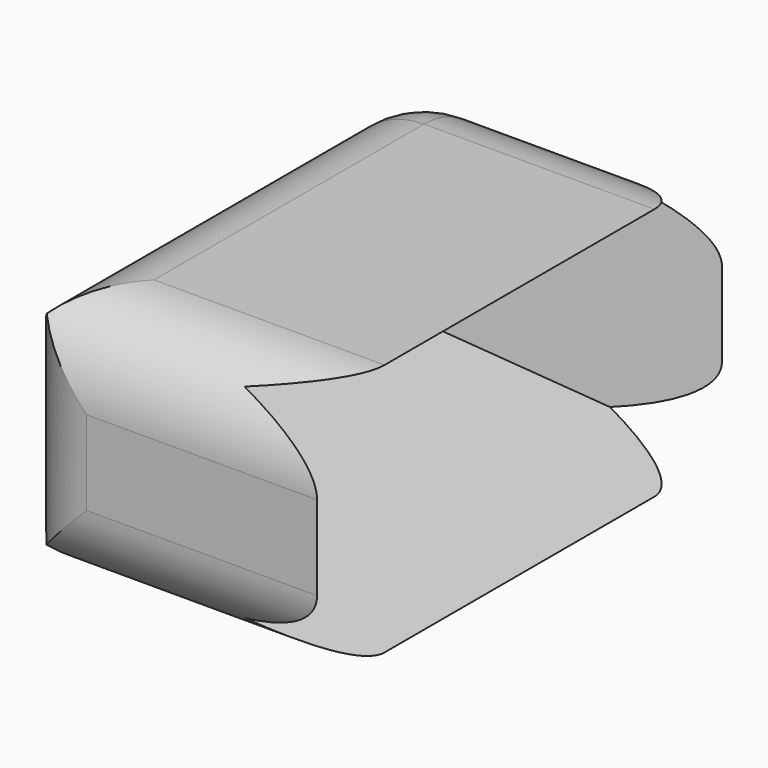
from build123d import *

# Parameters (mm, degrees)
F0_W         = 50
F0_H         = 15
F1_DEPTH     = 30
F2_R         = 5
F3_T1_DEPTH  = 52.5
F3_T3_DEPTH  = 5
F3_T5_DEPTH  = 32.5
F3_S9_W      = 5.1
F3_S9_H      = 5.1
F3_T10_DEPTH = 5.1
F3_S15_W     = 5.1
F3_S15_H     = 5.1
F3_T16_DEPTH = 5.1
F4_DEPTH     = 20
F1_FACE1_W   = 20
F1_FACE1_H   = 5
F5_DEPTH     = 57.6854757965
F5_TAPER     = -15


# Not quite as in the source:
# - a fillet or chamfer that OpenCascade refuses, or shapes differently, is made with other operations: its cross-section is extruded or revolved along the edge and cut away or added


with BuildPart() as f1:
    # F0 (on Front) → F1 (new body)
    with BuildSketch(Plane.XZ):
        with Locations((-8.187652571, -9.1238242388)):
            Rectangle(F0_W, F0_H)
    extrude(amount=F1_DEPTH)

    # F2
    f2_edges = [f1.edges().sort_by_distance(p)[0] for p in [
        (16.812347, -15, -16.623824),
        (16.812347, -15, -1.623824),
        (16.812347, 0, -9.123824),
        (16.812347, -30, -9.123824),
        (-8.187653, -30, -16.623824),
        (-8.187653, -30, -1.623824),
        (-33.187653, -30, -9.123824),
    ]]
    fillet(f2_edges, radius=F2_R)

    # F3: fillet of radius 5 on 7 edges, made by hand

    # F3_s2 → F3_t1 (cut)
    with BuildSketch(Plane.YZ.offset(-28.187652571)):
        with BuildLine():
            ThreePointArc((-5, -16.6238242388), (-1.4644660941, -15.1593581447), (0, -11.6238242388))
            Line((0, -11.6238242388), (0, -16.6238242388))
            Line((0, -16.6238242388), (-5, -16.6238242388))
        make_face()
        with BuildLine():
            ThreePointArc((0, -6.6238242388), (-1.4644660941, -3.0882903328), (-5, -1.6238242388))
            Line((-5, -1.6238242388), (0, -1.6238242388))
            Line((0, -1.6238242388), (0, -6.6238242388))
        make_face()
    extrude(amount=F3_T1_DEPTH, mode=Mode.SUBTRACT)

    # F3_s4 → F3_t3 (cut)
    with BuildSketch(Plane.XY.offset(-11.6238242388)):
        with BuildLine():
            ThreePointArc((-33.187652571, -5), (-31.7231864769, -1.4644660941), (-28.187652571, 0))
            Line((-28.187652571, 0), (-33.187652571, 0))
            Line((-33.187652571, 0), (-33.187652571, -5))
        make_face()
    extrude(amount=F3_T3_DEPTH, mode=Mode.SUBTRACT)

    # F3_s6 → F3_t5 (cut)
    with BuildSketch(Plane.XZ.offset(5)):
        with BuildLine():
            ThreePointArc((-33.187652571, -6.6238242388), (-31.7231864769, -3.0882903328), (-28.187652571, -1.6238242388))
            Line((-28.187652571, -1.6238242388), (-33.187652571, -1.6238242388))
            Line((-33.187652571, -1.6238242388), (-33.187652571, -6.6238242388))
        make_face()
        with BuildLine():
            ThreePointArc((-28.187652571, -16.6238242388), (-31.7231864769, -15.1593581447), (-33.187652571, -11.6238242388))
            Line((-33.187652571, -11.6238242388), (-33.187652571, -16.6238242388))
            Line((-33.187652571, -16.6238242388), (-28.187652571, -16.6238242388))
        make_face()
    extrude(amount=F3_T5_DEPTH, mode=Mode.SUBTRACT)


with BuildPart() as f3_tool8:
    # F3_s9 → F3_t10 (new body)
    with BuildSketch(Plane.XY.offset(-11.6238242388)):
        with Locations((-30.737652571, -2.45)):
            Rectangle(F3_S9_W, F3_S9_H)
    extrude(amount=-F3_T10_DEPTH)

    # F3_s11 → F3_t12 (revolve, cut)
    with BuildSketch(Plane(origin=(-28.187652571, -5, -11.6238242388), x_dir=(0.7071067812, -0.7071067812, 0), z_dir=(0.7071067812, 0.7071067812, 0))):
        with BuildLine():
            ThreePointArc((0, -5), (5, 0), (0, 5))
            Line((0, 5), (0, -5))
        make_face()
    revolve(axis=Axis((-28.187652571, -5, -11.6238242388), (0, 0, -1)), mode=Mode.SUBTRACT)


with BuildPart() as f1_1:
    add(f1.part)

    # F3_t7: cut F3_tool8
    add(f3_tool8.part, mode=Mode.SUBTRACT)


with BuildPart() as f3_tool14:
    # F3_s15 → F3_t16 (new body)
    with BuildSketch(Plane.YZ.offset(-28.187652571)):
        with Locations((-2.45, -4.0738242388)):
            Rectangle(F3_S15_W, F3_S15_H)
    extrude(amount=-F3_T16_DEPTH)

    # F3_s17 → F3_t18 (revolve, cut)
    with BuildSketch(Plane(origin=(-28.187652571, -5, -6.6238242388), x_dir=(0, -0.7071067812, -0.7071067812), z_dir=(0, 0.7071067812, -0.7071067812))):
        with BuildLine():
            ThreePointArc((0, -5), (5, 0), (0, 5))
            Line((0, 5), (0, -5))
        make_face()
    revolve(axis=Axis((-28.187652571, -5, -6.6238242388), (-1, 0, 0)), mode=Mode.SUBTRACT)


with BuildPart() as f1_2:
    add(f1_1.part)

    # F3_t13: cut F3_tool14
    add(f3_tool14.part, mode=Mode.SUBTRACT)

    # F4 (cut): a face of the model
    f4_faces = [f1_2.faces().sort_by_distance(p)[0] for p in [
        (16.812347429, -15, -9.1238242388),
    ]]
    extrude(f4_faces, amount=-F4_DEPTH, mode=Mode.SUBTRACT)

    # F1_face1 (on face) → F5 (cut)
    with BuildSketch(Plane(origin=(-33.187652571, -15, -9.1238242388), x_dir=(0, -1, 0), z_dir=(-1, 0, 0))):
        Rectangle(F1_FACE1_W, F1_FACE1_H)
    extrude(amount=-F5_DEPTH, taper=F5_TAPER, mode=Mode.SUBTRACT)


solid = f1_2.part
